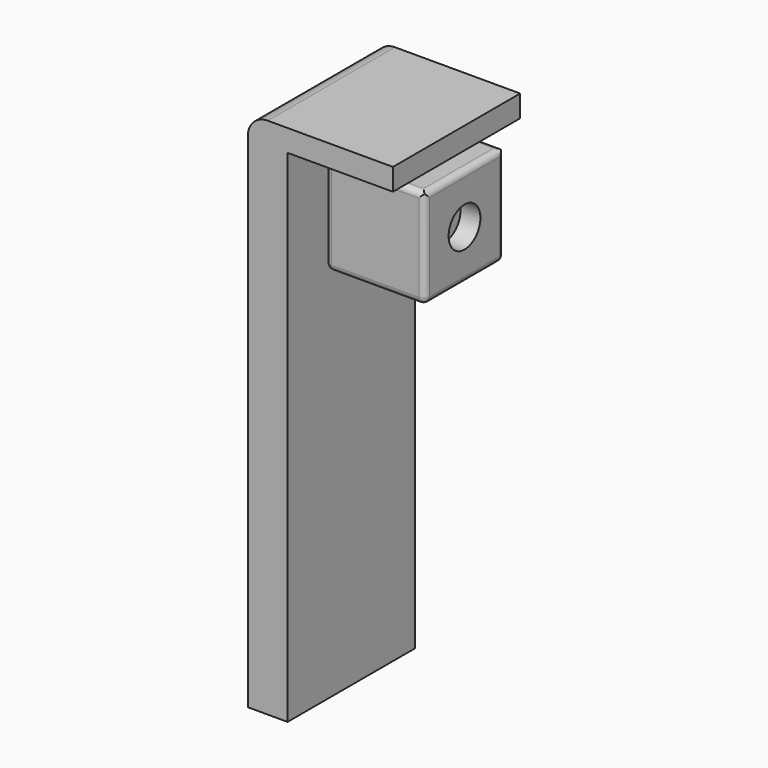
from build123d import *

# Parameters (mm, degrees)
F0_W           = 50
F0_H           = 50
F1_DEPTH       = 50
F2_R           = 3
F3_T1_DEPTH    = 51.5
F3_T3_DEPTH    = 44
F3_T5_DEPTH    = 44
F3_S9_W        = 3.06
F3_S9_H        = 3.06
F3_T10_DEPTH   = 3.06
F3_S15_W       = 3.06
F3_S15_H       = 3.06
F3_T16_DEPTH   = 3.06
F3_S21_W       = 3.06
F3_S21_H       = 3.06
F3_T22_DEPTH   = 3.06
F3_S27_W       = 3.06
F3_S27_H       = 3.06
F3_T28_DEPTH   = 3.06
F5_DEPTH       = 10
F6_R           = 10
F7_DEPTH       = 10
F4_R           = 10
F8_DEPTH       = 20
F10_DEPTH      = 40
F10_DEPTH_BACK = 40
F11_R          = 10


# Not quite as in the source:
# - a fillet or chamfer that OpenCascade refuses, or shapes differently, is made with other operations: its cross-section is extruded or revolved along the edge and cut away or added


with BuildPart() as f1:
    # F0 (on Top) → F1 (new body)
    with BuildSketch(Plane.XY):
        Rectangle(F0_W, F0_H)
    extrude(amount=F1_DEPTH)

    # F2
    f2_edges = [f1.edges().sort_by_distance(p)[0] for p in [
        (25, 0, 50),
        (0, 25, 50),
        (-25, 0, 50),
        (0, -25, 50),
    ]]
    fillet(f2_edges, radius=F2_R)

    # F3: fillet of radius 3 on 12 edges, made by hand

    # F3_s2 → F3_t1 (cut)
    with BuildSketch(Plane.XY.offset(3)):
        with BuildLine():
            ThreePointArc((-22, -25), (-24.1213203436, -24.1213203436), (-25, -22))
            Line((-25, -22), (-25, -25))
            Line((-25, -25), (-22, -25))
        make_face()
        with BuildLine():
            ThreePointArc((25, -22), (24.1213203436, -24.1213203436), (22, -25))
            Line((22, -25), (25, -25))
            Line((25, -25), (25, -22))
        make_face()
        with BuildLine():
            ThreePointArc((25, 22), (24.1213203436, 24.1213203436), (22, 25))
            Line((22, 25), (25, 25))
            Line((25, 25), (25, 22))
        make_face()
        with BuildLine():
            ThreePointArc((-22, 25), (-24.1213203436, 24.1213203436), (-25, 22))
            Line((-25, 22), (-25, 25))
            Line((-25, 25), (-22, 25))
        make_face()
    extrude(amount=F3_T1_DEPTH, mode=Mode.SUBTRACT)

    # F3_s4 → F3_t3 (cut)
    with BuildSketch(Plane.YZ.offset(-22)):
        with BuildLine():
            ThreePointArc((-25, 3), (-24.1213203436, 0.8786796564), (-22, 0))
            Line((-22, 0), (-25, 0))
            Line((-25, 0), (-25, 3))
        make_face()
        with BuildLine():
            ThreePointArc((22, 0), (24.1213203436, 0.8786796564), (25, 3))
            Line((25, 3), (25, 0))
            Line((25, 0), (22, 0))
        make_face()
    extrude(amount=F3_T3_DEPTH, mode=Mode.SUBTRACT)

    # F3_s6 → F3_t5 (cut)
    with BuildSketch(Plane.XZ.offset(-22)):
        with BuildLine():
            ThreePointArc((25, 3), (24.1213203436, 0.8786796564), (22, 0))
            Line((22, 0), (25, 0))
            Line((25, 0), (25, 3))
        make_face()
        with BuildLine():
            ThreePointArc((-22, 0), (-24.1213203436, 0.8786796564), (-25, 3))
            Line((-25, 3), (-25, 0))
            Line((-25, 0), (-22, 0))
        make_face()
    extrude(amount=F3_T5_DEPTH, mode=Mode.SUBTRACT)


with BuildPart() as f3_tool8:
    # F3_s9 → F3_t10 (new body)
    with BuildSketch(Plane.XZ.offset(22)):
        with Locations((-23.53, 1.47)):
            Rectangle(F3_S9_W, F3_S9_H)
    extrude(amount=F3_T10_DEPTH)

    # F3_s11 → F3_t12 (revolve, cut)
    with BuildSketch(Plane(origin=(-22, -22, 3), x_dir=(0.7071067812, 0, 0.7071067812), z_dir=(0.7071067812, 0, -0.7071067812))):
        with BuildLine():
            ThreePointArc((0, -3), (3, 0), (0, 3))
            Line((0, 3), (0, -3))
        make_face()
    revolve(axis=Axis((-22, -22, 3), (0, -1, 0)), mode=Mode.SUBTRACT)


with BuildPart() as f1_1:
    add(f1.part)

    # F3_t7: cut F3_tool8
    add(f3_tool8.part, mode=Mode.SUBTRACT)


with BuildPart() as f3_tool14:
    # F3_s15 → F3_t16 (new body)
    with BuildSketch(Plane.YZ.offset(22)):
        with Locations((-23.53, 1.47)):
            Rectangle(F3_S15_W, F3_S15_H)
    extrude(amount=F3_T16_DEPTH)

    # F3_s17 → F3_t18 (revolve, cut)
    with BuildSketch(Plane(origin=(22, -22, 3), x_dir=(0, 0.7071067812, 0.7071067812), z_dir=(0, 0.7071067812, -0.7071067812))):
        with BuildLine():
            ThreePointArc((0, -3), (3, 0), (0, 3))
            Line((0, 3), (0, -3))
        make_face()
    revolve(axis=Axis((22, -22, 3), (1, 0, 0)), mode=Mode.SUBTRACT)


with BuildPart() as f1_2:
    add(f1_1.part)

    # F3_t13: cut F3_tool14
    add(f3_tool14.part, mode=Mode.SUBTRACT)


with BuildPart() as f3_tool20:
    # F3_s21 → F3_t22 (new body)
    with BuildSketch(Plane.YZ.offset(22)):
        with Locations((23.53, 1.47)):
            Rectangle(F3_S21_W, F3_S21_H)
    extrude(amount=F3_T22_DEPTH)

    # F3_s23 → F3_t24 (revolve, cut)
    with BuildSketch(Plane(origin=(22, 22, 3), x_dir=(0, -0.7071067812, 0.7071067812), z_dir=(0, 0.7071067812, 0.7071067812))):
        with BuildLine():
            ThreePointArc((0, -3), (3, 0), (0, 3))
            Line((0, 3), (0, -3))
        make_face()
    revolve(axis=Axis((22, 22, 3), (1, 0, 0)), mode=Mode.SUBTRACT)


with BuildPart() as f1_3:
    add(f1_2.part)

    # F3_t19: cut F3_tool20
    add(f3_tool20.part, mode=Mode.SUBTRACT)


with BuildPart() as f3_tool26:
    # F3_s27 → F3_t28 (new body)
    with BuildSketch(Plane.XY.offset(3)):
        with Locations((-23.53, 23.53)):
            Rectangle(F3_S27_W, F3_S27_H)
    extrude(amount=-F3_T28_DEPTH)

    # F3_s29 → F3_t30 (revolve, cut)
    with BuildSketch(Plane(origin=(-22, 22, 3), x_dir=(0.7071067812, -0.7071067812, 0), z_dir=(0.7071067812, 0.7071067812, 0))):
        with BuildLine():
            ThreePointArc((0, -3), (3, 0), (0, 3))
            Line((0, 3), (0, -3))
        make_face()
    revolve(axis=Axis((-22, 22, 3), (0, 0, -1)), mode=Mode.SUBTRACT)


with BuildPart() as f1_4:
    add(f1_3.part)

    # F3_t25: cut F3_tool26
    add(f3_tool26.part, mode=Mode.SUBTRACT)

    # F5 (cut): a face of the model
    f5_faces = [f1_4.faces().sort_by_distance(p)[0] for p in [
        (0, 0, 0),
    ]]
    extrude(f5_faces, amount=-F5_DEPTH, mode=Mode.SUBTRACT)

    # F6 (on face) → F7 (cut)
    with BuildSketch(Plane.YZ.offset(25)):
        with Locations((0, 25)):
            Circle(F6_R)
    extrude(amount=-F7_DEPTH, mode=Mode.SUBTRACT)

    # F4 (on face) → F8 (join)
    with BuildSketch(Plane(origin=(-25, 0, 0), x_dir=(0, -1, 0), z_dir=(-1, 0, 0))):
        with Locations((0, 25)):
            Circle(F4_R)
    extrude(amount=F8_DEPTH)

    # F9 (on Front) → F10 (join, two sides)
    with BuildSketch(Plane.XZ) as f10_sk:
        Polygon((21, 55.5713325143), (21, 66.5713325143), (-52, 66.5713325143), (-52, -196.4604258537), (-32, -196.4604258537), (-32, 55.5713325143), align=None)
    extrude(amount=F10_DEPTH)
    extrude(f10_sk.sketch, amount=-F10_DEPTH_BACK)

    # F11
    f11_edges = [f1_4.edges().sort_by_distance(p)[0] for p in [
        (-52, 0, 66.571333),
    ]]
    fillet(f11_edges, radius=F11_R)


solid = f1_4.part
